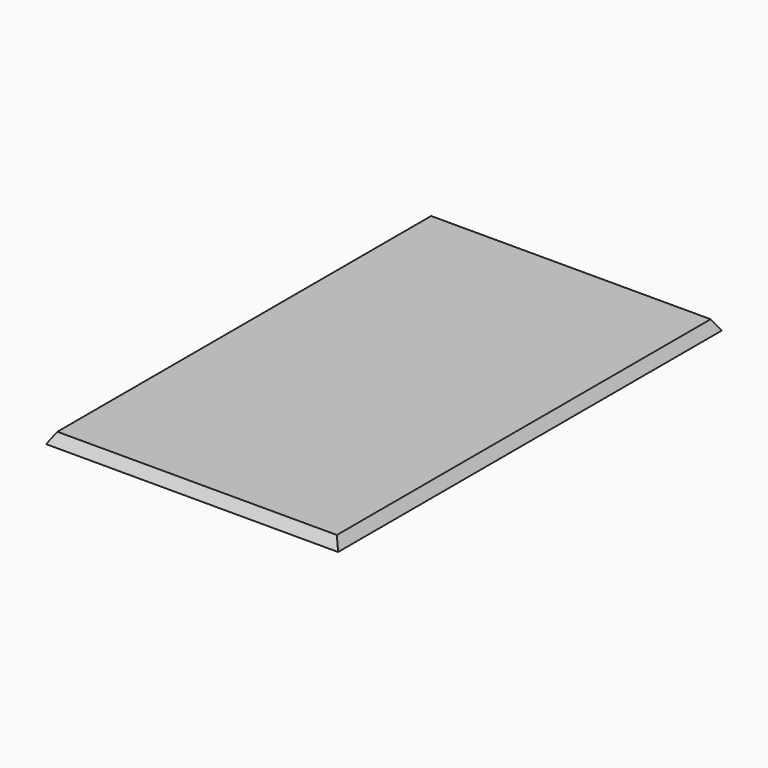
from build123d import *

# Parameters (mm, degrees)
F0_W     = 1400
F0_H     = 2300
F1_DEPTH = 50
F2_SIZE2 = 49.99999
F2_SIZE  = 29.99999


# Not quite as in the source:
# - a fillet or chamfer is up to 0.001 mm smaller than in the source, because OpenCascade refuses the exact size


with BuildPart() as f1:
    # F0 (on Top) → F1 (new body)
    with BuildSketch(Plane.XY):
        Rectangle(F0_W, F0_H)
    extrude(amount=F1_DEPTH)

    # F2 (size 30 and 50 in the source; OpenCascade refuses exactly that, so slightly less here)
    f2_edges = [f1.edges().sort_by_distance(p)[0] for p in [
        (0, -1150, 50),
        (700, 0, 50),
        (0, 1150, 50),
        (-700, 0, 50),
    ]]
    f2_side = f1.faces().sort_by_distance((0, 0, 50))[0]
    chamfer(f2_edges, length=F2_SIZE, length2=F2_SIZE2, reference=f2_side)


solid = f1.part
